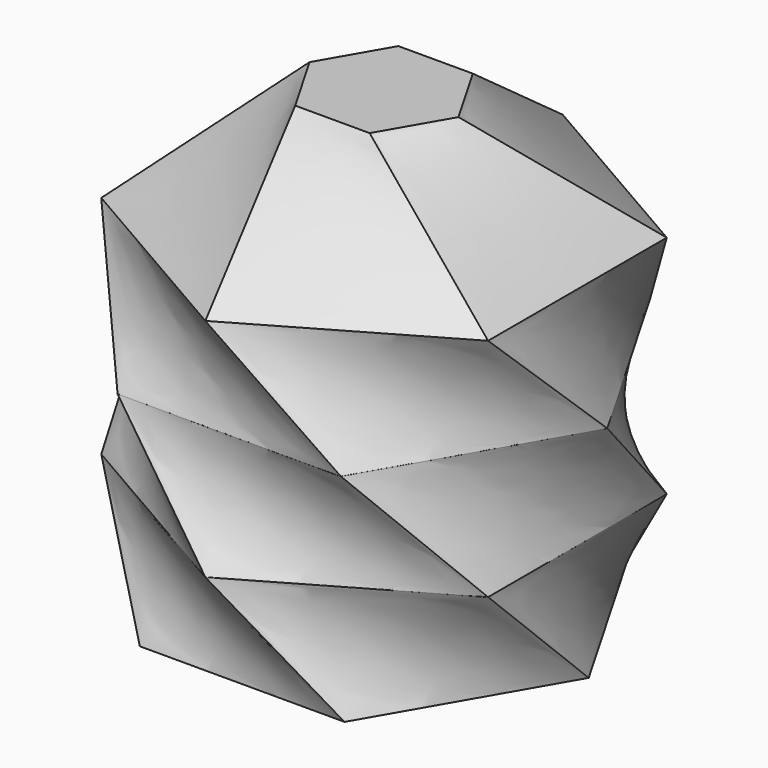
from build123d import *


with BuildPart() as f9:
    # F4 (on Top) → F9 section 0
    with BuildSketch(Plane.XY):
        Polygon((-31.754265, -55), (31.754265, -55), (63.50853, 0), (31.754265, 55), (-31.754265, 55), (-63.50853, 0), align=None)
    # F5 (on offset) → F9 section 1
    with BuildSketch(Plane.XY.offset(35)):
        Polygon((60, -34.641016), (60, 34.641016), (0, 69.282032), (-60, 34.641016), (-60, -34.641016), (0, -69.282032), align=None)
    loft()

    # F5 (on offset) → F10 section 0
    with BuildSketch(Plane.XY.offset(35)):
        Polygon((60, -34.641016), (60, 34.641016), (0, 69.282032), (-60, 34.641016), (-60, -34.641016), (0, -69.282032), align=None)
    # F6 (on offset) → F10 section 1
    with BuildSketch(Plane.XY.offset(70)):
        Polygon((34.641016, -60), (69.282032, 0), (34.641016, 60), (-34.641016, 60), (-69.282032, 0), (-34.641016, -60), align=None)
    loft()

    # F6 (on offset) → F11 section 0
    with BuildSketch(Plane.XY.offset(70)):
        Polygon((34.641016, -60), (69.282032, 0), (34.641016, 60), (-34.641016, 60), (-69.282032, 0), (-34.641016, -60), align=None)
    # F7 (on offset) → F11 section 1
    with BuildSketch(Plane.XY.offset(105)):
        Polygon((0, -69.282032), (60, -34.641016), (60, 34.641016), (0, 69.282032), (-60, 34.641016), (-60, -34.641016), align=None)
    loft()

    # F7 (on offset) → F12 section 0
    with BuildSketch(Plane.XY.offset(105)):
        Polygon((0, -69.282032), (60, -34.641016), (60, 34.641016), (0, 69.282032), (-60, 34.641016), (-60, -34.641016), align=None)
    # F8 (on offset) → F12 section 1
    with BuildSketch(Plane.XY.offset(140)):
        Polygon((11.547005, -20), (23.094011, 0), (11.547005, 20), (-11.547005, 20), (-23.094011, 0), (-11.547005, -20), align=None)
    loft()


solid = f9.part
